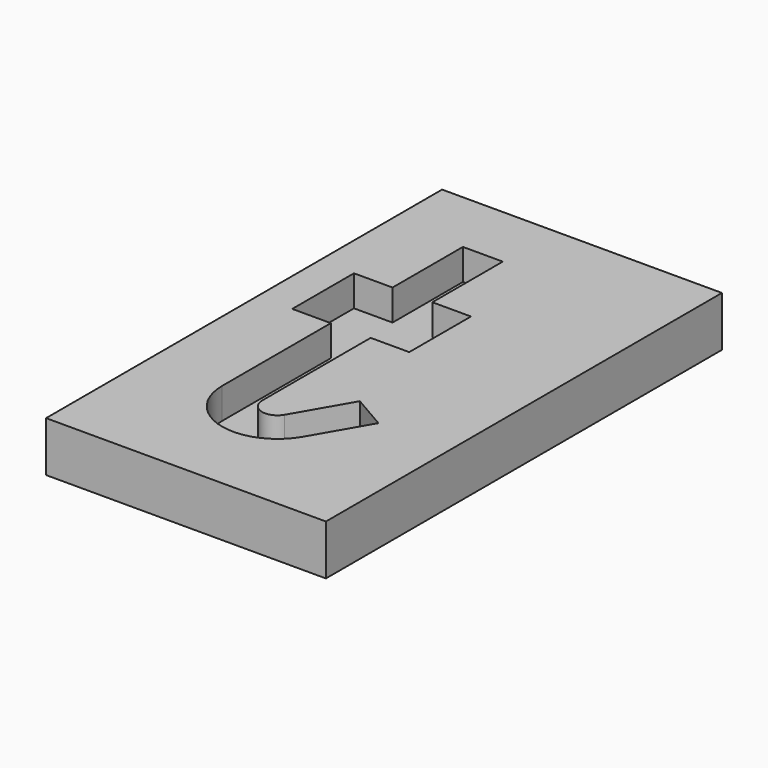
from build123d import *

# Parameters (mm, degrees)
F0_W     = 72.546231
F0_H     = 128.329664
F1_DEPTH = 13
F3_DEPTH = 8


# Not quite as in the source:
# - ends of sketch curves that miss each other by under 0.0002 mm in the source are joined


with BuildPart() as f1:
    # F0 (on Top) → F1 (new body)
    with BuildSketch(Plane.XY):
        with Locations((5e-07, 0)):
            Rectangle(F0_W, F0_H)
    extrude(amount=F1_DEPTH)

    # F2 (on face) → F3 (cut)
    with BuildSketch(Plane.XY.offset(13)):
        with BuildLine():
            Line((-6.941915, 24.355961), (-6.941915, 47.164832))
            Line((-6.941915, 47.164832), (-17.273115, 47.164832))
            Line((-17.273115, 47.164832), (-17.273115, 24.355961))
            Line((-17.273115, 24.355961), (-27.273115, 24.355961))
            Line((-27.273115, 24.355961), (-27.273115, 4.355961))
            Line((-27.273115, 4.355961), (-17.273115, 4.355961))
            Line((-17.273115, 4.355961), (-17.2731146267, -30.8336322155))
            Line((-17.2731146267, -30.8336322155), (-17.2731146267, -30.8377282155))
            Line((-17.2731146267, -30.8377282155), (-17.2731139504, -30.8380352155))
            ThreePointArc((-17.2731139504, -30.8380352155), (-6.6489757762, -44.6770778186), (9.4692682, -37.9992321155))
            Line((9.4692682, -37.9992321155), (17.6391412, -23.8485971155))
            Line((17.6391412, -23.8485971155), (8.69206, -18.682997))
            Line((8.69206, -18.682997), (0.522187, -32.833632))
            ThreePointArc((0.522187, -32.833632), (-3.9764490293, -34.6975341769), (-6.9419144165, -30.8351679998))
            Line((-6.9419144165, -30.8351679998), (-6.94191496, -30.8348611666))
            Line((-6.94191496, -30.8348611666), (-6.94191496, -30.8336322155))
            Line((-6.94191496, -30.8336322155), (-6.94191496, 4.355961))
            Line((-6.94191496, 4.355961), (3.058085, 4.355961))
            Line((3.058085, 4.355961), (3.05808504, 24.355961))
            Line((3.05808504, 24.355961), (-6.941915, 24.355961))
        make_face()
    extrude(amount=-F3_DEPTH, mode=Mode.SUBTRACT)


solid = f1.part
